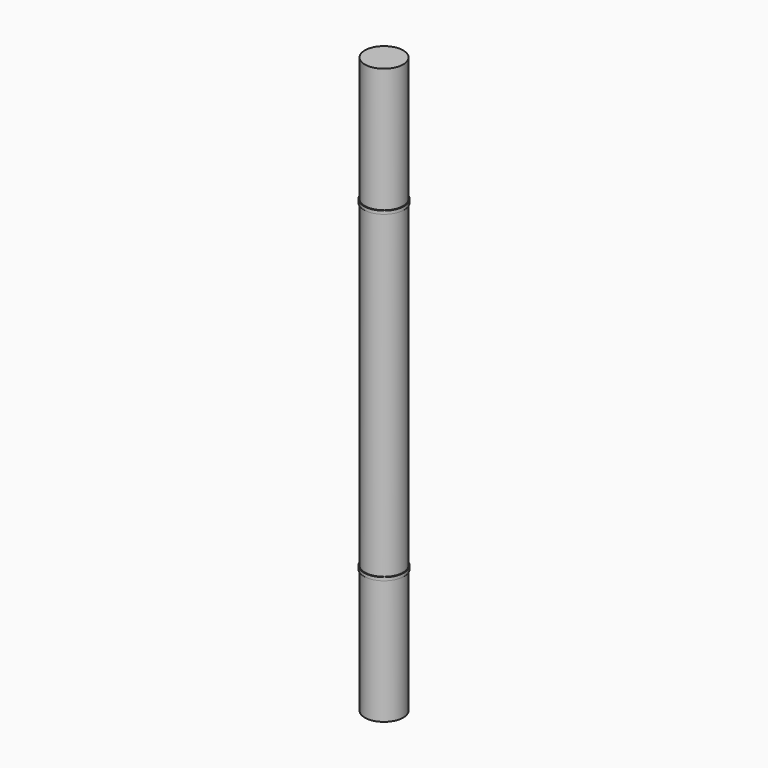
from build123d import *

# Parameters (mm, degrees)
F0_R     = 60
F1_DEPTH = 900
F4_R     = 62.5
F4_R_2   = 60
F5_DEPTH = 10


# Not quite as in the source:
# - a pattern or mirror of a feature is missing from the dataset's text; its kind, count and spacing are read off the source's solid


with BuildPart() as f1:
    # F0 (on Top) → F1 (new body)
    with BuildSketch(Plane.XY):
        Circle(F0_R)
    extrude(amount=F1_DEPTH)

    # F2: F1 across plane


with BuildPart() as f1_1:
    add(f1.part)
    add(f1.part.mirror(Plane.XY))

    # F4 (on offset) → F5 (join)
    with BuildSketch(Plane.XY.offset(500)):
        Circle(F4_R)
        Circle(F4_R_2, mode=Mode.SUBTRACT)
    f5 = extrude(amount=F5_DEPTH)

    # F5_copies: F5 across plane
    add(f5.mirror(Plane(origin=(0, 0, 0), x_dir=(-1, 0, 0), z_dir=(0, 0, -1))))


solid = f1_1.part
